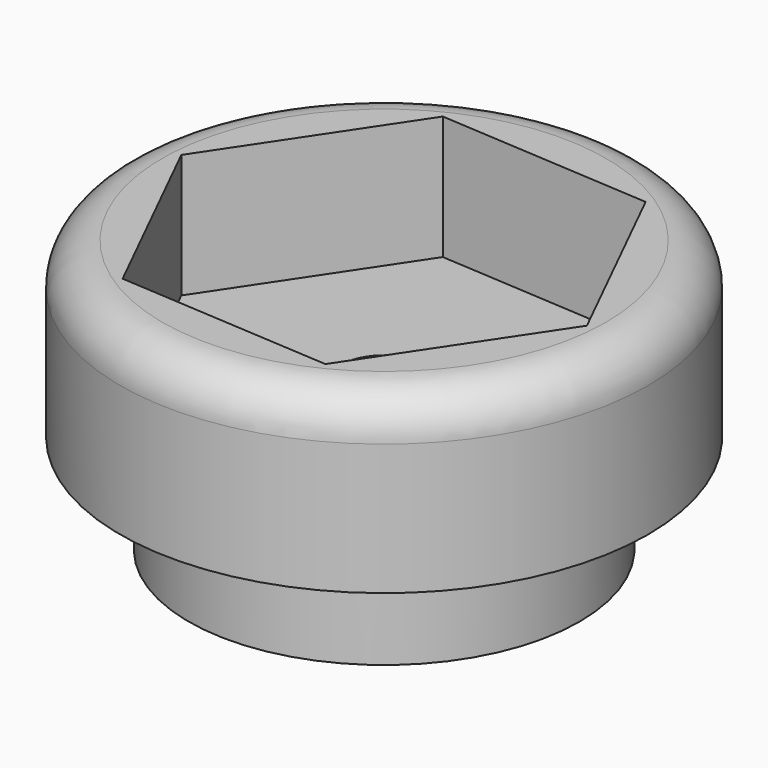
from build123d import *
from build123d import SkipClean  # not in build123d's __all__

# Parameters (mm, degrees)
F0_R      = 10.668
F1_DEPTH  = 7
F4_DEPTH  = 2
F7_DEPTH  = 2
F8_R      = 7.8995
F9_DEPTH  = 6
F5_R      = 1.75
F10_DEPTH = 25
F11_R     = 1.7


with BuildPart() as f1:
    # F0 (on Top) → F1 (new body)
    with BuildSketch(Plane.XY):
        Circle(F0_R)
        Polygon((-4.8043411611, -7.2054358652), (-8.6422610852, 0.5579635614), (-3.837919924, 7.7633994266), (4.8043411611, 7.2054358652), (8.6422610852, -0.5579635614), (3.837919924, -7.7633994266), align=None, mode=Mode.SUBTRACT)
    extrude(amount=F1_DEPTH)

    # F3 (on offset) → F4 (join)
    with BuildSketch(Plane(origin=(0, 0, 2), x_dir=(1, 0, 0), z_dir=(0, 0, -1))):
        with BuildLine():
            ThreePointArc((1.9919788729, 7.6442213744), (3.5007804976, 7.081428963), (4.8641016704, 6.2243566085))
            Line((4.8641016704, 6.2243566085), (3.837919924, 7.7633994266))
            Line((3.837919924, 7.7633994266), (1.9919788729, 7.6442213744))
        make_face()
        with BuildLine():
            ThreePointArc((-5.6241004659, 5.5472149949), (-4.3823071282, 6.5724793255), (-2.95840011, 7.3246139174))
            Line((-2.95840011, 7.3246139174), (-4.8043411611, 7.2054358652))
            Line((-4.8043411611, 7.2054358652), (-5.6241004659, 5.5472149949))
        make_face()
        with BuildLine():
            ThreePointArc((-7.6160793388, -2.0970063795), (-7.8830876258, -0.5089496375), (-7.8225017804, 1.1002573089))
            Line((-7.8225017804, 1.1002573089), (-8.6422610852, -0.5579635614))
            Line((-8.6422610852, -0.5579635614), (-7.6160793388, -2.0970063795))
        make_face()
        with BuildLine():
            Line((-3.837919924, -7.7633994266), (-1.9919788729, -7.6442213744))
            ThreePointArc((-1.9919788729, -7.6442213744), (-3.5007804976, -7.081428963), (-4.8641016704, -6.2243566085))
            Line((-4.8641016704, -6.2243566085), (-3.837919924, -7.7633994266))
        make_face()
        with BuildLine():
            ThreePointArc((7.6160793388, 2.0970063795), (7.8283241817, 1.0580362738), (7.8995, 0))
            ThreePointArc((7.8995, 0), (7.880226934, -0.5514741317), (7.8225017804, -1.1002573089))
            Line((7.8225017804, -1.1002573089), (8.6422610852, 0.5579635614))
            Line((8.6422610852, 0.5579635614), (7.6160793388, 2.0970063795))
        make_face()
        with BuildLine():
            Line((4.8043411611, -7.2054358652), (5.6241004659, -5.5472149949))
            ThreePointArc((5.6241004659, -5.5472149949), (4.3823071282, -6.5724793255), (2.95840011, -7.3246139174))
            Line((2.95840011, -7.3246139174), (4.8043411611, -7.2054358652))
        make_face()
    extrude(amount=F4_DEPTH)

    # F6 (on face) → F7 (cut)
    with BuildSketch(Plane(origin=(0, 0, 0), x_dir=(1, 0, 0), z_dir=(0, 0, -1))):
        with BuildLine():
            Line((4.8641016704, 6.2243566085), (7.6160793388, 2.0970063795))
            ThreePointArc((7.6160793388, 2.0970063795), (6.5724793255, 4.3823071282), (4.8641016704, 6.2243566085))
        make_face()
        with BuildLine():
            ThreePointArc((5.6241004659, -5.5472149949), (7.081428963, -3.5007804976), (7.8225017804, -1.1002573089))
            Line((7.8225017804, -1.1002573089), (5.6241004659, -5.5472149949))
        make_face()
        with BuildLine():
            ThreePointArc((-1.9919788729, -7.6442213744), (0.5089496375, -7.8830876258), (2.95840011, -7.3246139174))
            Line((2.95840011, -7.3246139174), (-1.9919788729, -7.6442213744))
        make_face()
        with BuildLine():
            ThreePointArc((-7.6160793388, -2.0970063795), (-6.5724793255, -4.3823071282), (-4.8641016704, -6.2243566085))
            Line((-4.8641016704, -6.2243566085), (-7.6160793388, -2.0970063795))
        make_face()
        with BuildLine():
            Line((-7.8225017804, 1.1002573089), (-5.6241004659, 5.5472149949))
            ThreePointArc((-5.6241004659, 5.5472149949), (-7.081428963, 3.5007804976), (-7.8225017804, 1.1002573089))
        make_face()
        with BuildLine():
            Line((-2.95840011, 7.3246139174), (1.9919788729, 7.6442213744))
            ThreePointArc((1.9919788729, 7.6442213744), (-0.5089496375, 7.8830876258), (-2.95840011, 7.3246139174))
        make_face()
    with SkipClean():  # cleaning this boolean's faces spoils the solid; the shape is the same uncleaned
        extrude(amount=-F7_DEPTH, mode=Mode.SUBTRACT)

    # F8 (on offset) → F9 (join)
    with BuildSketch(Plane(origin=(0, 0, 2), x_dir=(1, 0, 0), z_dir=(0, 0, -1))):
        Circle(F8_R)
    extrude(amount=F9_DEPTH)

    # F5 (on face) → F10 (cut)
    with BuildSketch(Plane.XY.offset(2)):
        Circle(F5_R)
    extrude(amount=-F10_DEPTH, mode=Mode.SUBTRACT)

    # F11
    f11_edges = [f1.edges().sort_by_distance(p)[0] for p in [
        (-10.668, 0, 7),
    ]]
    fillet(f11_edges, radius=F11_R)


solid = f1.part
